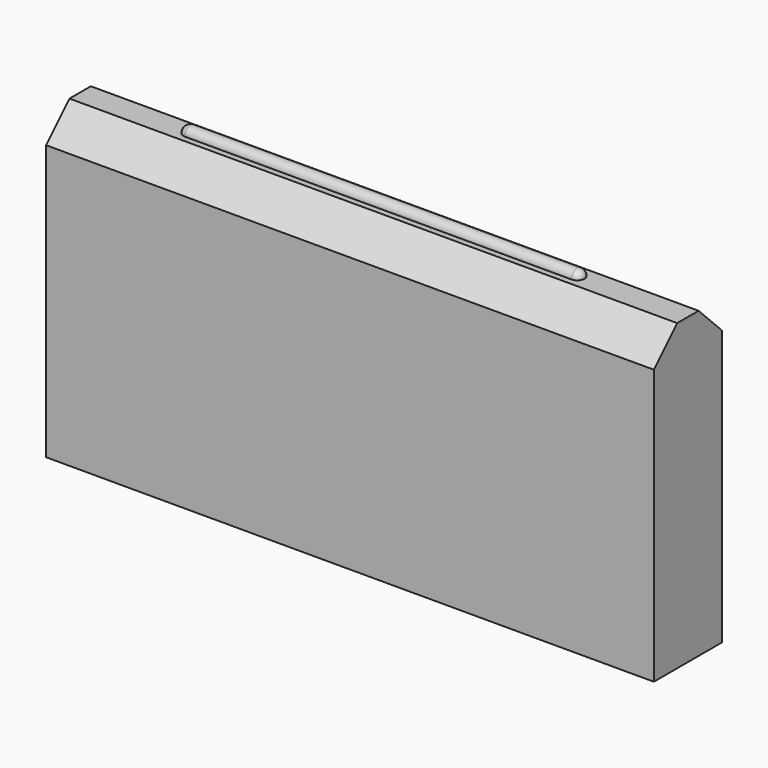
from build123d import *

# Parameters (mm, degrees)
F0_W     = 50
F0_H     = 7
F1_DEPTH = 25
F2_SIZE  = 2.4
F3_R     = 0.6
F4_DEPTH = 16.5
F5_R     = 0.59999


# Not quite as in the source:
# - a fillet or chamfer is up to 0.001 mm smaller than in the source, because OpenCascade refuses the exact size


with BuildPart() as f1:
    # F0 (on Top) → F1 (new body)
    with BuildSketch(Plane.XY):
        Rectangle(F0_W, F0_H)
    extrude(amount=F1_DEPTH)

    # F2
    f2_edges = [f1.edges().sort_by_distance(p)[0] for p in [
        (0, -3.5, 25),
        (0, 3.5, 25),
    ]]
    chamfer(f2_edges, length=F2_SIZE)

    # F3 (on Right) → F4 (join, symmetric)
    with BuildSketch(Plane.YZ):
        with Locations((0, 25)):
            Circle(F3_R)
    extrude(amount=F4_DEPTH, both=True)

    # F5 (radius 0.6 in the source; OpenCascade refuses exactly that, so slightly less here)
    f5_edges = [f1.edges().sort_by_distance(p)[0] for p in [
        (16.5, 0, 25.6),
        (-16.5, 0, 25.6),
    ]]
    fillet(f5_edges, radius=F5_R)


solid = f1.part
